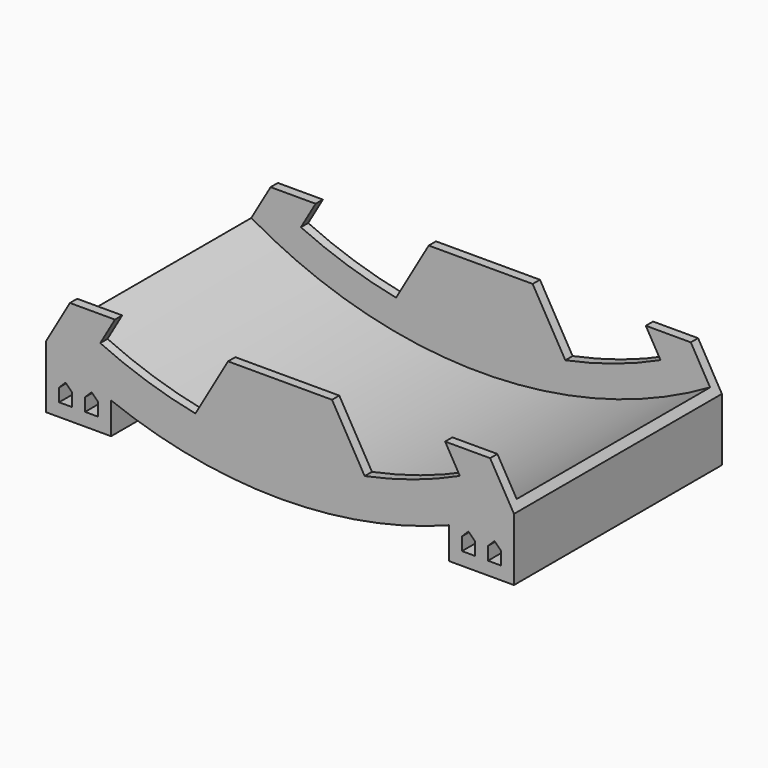
from build123d import *

# Parameters (mm, degrees)
F1_DEPTH  = 127
F2_T      = 4.445
F3_R      = 9.525
F4_DEPTH  = 127
F6_DEPTH  = 127
F8_DEPTH  = 154.94
F10_DEPTH = 4.445
F14_DEPTH = 127


# Not quite as in the source:
# - a shell that OpenCascade refuses in one call is made with other operations: the cavity is built on its own and cut out


with BuildPart() as f1:
    # F0 (on Front) → F1 (new body)
    with BuildSketch(Plane.XZ):
        with BuildLine():
            Line((-19.05, -32.9955678842), (-114.3, -197.9734073051))
            ThreePointArc((-114.3, -197.9734073051), (0, -228.6), (114.3, -197.9734073051))
            Line((114.3, -197.9734073051), (19.05, -32.9955678842))
            ThreePointArc((19.05, -32.9955678842), (32.9955678842, -19.05), (38.1, 0))
            ThreePointArc((38.1, 0), (0, 38.1), (-38.1, 0))
            ThreePointArc((-38.1, 0), (-32.9955678842, -19.05), (-19.05, -32.9955678842))
        make_face()
    extrude(amount=F1_DEPTH)

    # F2: shell of thickness 4.445, made by hand


with BuildPart() as f2_core1:
    # F2_t2: copy of F1
    add(f1.part)

    # the walls: a layer under each face that stays
    f2_faces = [f2_core1.faces().sort_by_distance(p)[0] for p in [
        (0, -127, -95.25),
        (0, 0, -95.25),
        (0, -63.5, -228.6),
        (-32.9955678842, -63.5, -19.05),
    ]]
    thicken(f2_faces, amount=-F2_T, mode=Mode.SUBTRACT)


with BuildPart() as f1_1:
    add(f1.part)

    # what is left inside the walls is the cavity
    f2_cavity = [f2_core1.part.solids().sort_by_distance(p)[0] for p in [
        (0, -122.51055, -136.736667),
    ]]
    add(f2_cavity, mode=Mode.SUBTRACT)

    # F3 (on face) → F4 (cut, through all)
    with BuildSketch(Plane.XZ.offset(127)):
        with BuildLine():
            Line((-50.6196632626, -125.7758286329), (-87.8433632626, -190.2491682786))
            ThreePointArc((-87.8433632626, -190.2491682786), (-48.4057129805, -203.8825383667), (-7.0486462544, -209.4314185741))
            Line((-7.0486462544, -209.4314185741), (-7.0486462544, -169.3468456411))
            Line((-7.0486462544, -169.3468456411), (-50.6196632626, -125.7758286329))
        make_face()
        with BuildLine():
            Line((87.8433632626, -190.2491682786), (50.6196632626, -125.7758286329))
            Line((50.6196632626, -125.7758286329), (7.0486462544, -169.3468456411))
            Line((7.0486462544, -169.3468456411), (7.0486462544, -209.4314185741))
            ThreePointArc((7.0486462544, -209.4314185741), (48.4057129805, -203.8825383667), (87.8433632626, -190.2491682786))
        make_face()
        with BuildLine():
            Line((44.2696632626, -114.7773060049), (7.0486462544, -50.3086134373))
            Line((7.0486462544, -50.3086134373), (7.0486462544, -125.901221947))
            ThreePointArc((7.0486462544, -125.901221947), (11.356209976, -128.3041542134), (14.9024469628, -131.7324762409))
            Line((14.9024469628, -131.7324762409), (44.2696632626, -114.7773060049))
        make_face()
        with BuildLine():
            Line((-7.0486462544, -125.901221947), (-7.0486462544, -50.3086134373))
            Line((-7.0486462544, -50.3086134373), (-44.2696632626, -114.7773060049))
            Line((-44.2696632626, -114.7773060049), (-14.9024469628, -131.7324762409))
            ThreePointArc((-14.9024469628, -131.7324762409), (-11.356209976, -128.3041542134), (-7.0486462544, -125.901221947))
        make_face()
        Circle(F3_R)
    extrude(amount=-F4_DEPTH, mode=Mode.SUBTRACT)

    # F5 (on Front) → F6 (join, through all)
    with BuildSketch(Plane.XZ):
        with BuildLine():
            ThreePointArc((114.3, -197.9734073051), (59.1660337104, -220.8106438897), (0, -228.6))
            Line((0, -228.6), (114.3, -228.6))
            Line((114.3, -228.6), (114.3, -197.9734073051))
        make_face()
        Polygon((95.25, -222.25), (88.9, -222.25), (88.9, -215.9), (92.075, -212.725), (95.25, -215.9), align=None, mode=Mode.SUBTRACT)
        Polygon((107.95, -215.9), (107.95, -222.25), (101.6, -222.25), (101.6, -215.9), (104.775, -212.725), align=None, mode=Mode.SUBTRACT)
        with BuildLine():
            Line((-114.3, -228.6), (0, -228.6))
            ThreePointArc((0, -228.6), (-59.1660337104, -220.8106438897), (-114.3, -197.9734073051))
            Line((-114.3, -197.9734073051), (-114.3, -228.6))
        make_face()
        Polygon((-104.775, -212.725), (-101.6, -215.9), (-101.6, -222.25), (-107.95, -222.25), (-107.95, -215.9), align=None, mode=Mode.SUBTRACT)
        Polygon((-92.075, -212.725), (-88.9, -215.9), (-88.9, -222.25), (-95.25, -222.25), (-95.25, -215.9), align=None, mode=Mode.SUBTRACT)
    extrude(amount=F6_DEPTH)

    # F7 (on Front) → F8 (cut)
    with BuildSketch(Plane.XZ):
        Polygon((-155.1303118467, -177.8), (0, -177.8), (122.5007101893, -177.8), (122.5007101893, 99.952660501), (-155.1303118467, 97.6831391454), align=None)
    extrude(amount=F8_DEPTH, mode=Mode.SUBTRACT)

    # F9 (on face) → F10 (join, through all)
    with BuildSketch(Plane(origin=(0, 0, 0), x_dir=(-1, 0, 0), z_dir=(0, 1, 0))):
        with BuildLine():
            ThreePointArc((-41.3518280797, -205.4293767076), (-65.0419791249, -199.2002596673), (-87.8433632626, -190.2491682786))
            Line((-87.8433632626, -190.2491682786), (-80.6558326058, -177.8))
            Line((-80.6558326058, -177.8), (-102.6528778619, -177.8))
            Line((-102.6528778619, -177.8), (-114.3, -197.9734073051))
            Line((-114.3, -197.9734073051), (-114.3, -228.6))
            Line((-114.3, -228.6), (114.3, -228.6))
            Line((114.3, -228.6), (114.3, -197.9734073051))
            Line((114.3, -197.9734073051), (102.6528778619, -177.8))
            Line((102.6528778619, -177.8), (80.6558326058, -177.8))
            Line((80.6558326058, -177.8), (87.8433632626, -190.2491682786))
            ThreePointArc((87.8433632626, -190.2491682786), (65.0419791249, -199.2002596673), (41.3518280797, -205.4293767076))
            ThreePointArc((41.3518280797, -205.4293767076), (24.2828244592, -208.1382880113), (7.0486462544, -209.4314185741))
            Line((7.0486462544, -209.4314185741), (7.0486462544, -177.8))
            Line((7.0486462544, -177.8), (0, -177.8))
            Line((0, -177.8), (-7.0486462544, -177.8))
            Line((-7.0486462544, -177.8), (-7.0486462544, -209.4314185741))
            ThreePointArc((-7.0486462544, -209.4314185741), (-24.2828244592, -208.1382880113), (-41.3518280797, -205.4293767076))
        make_face()
        Polygon((-107.95, -222.25), (-107.95, -215.9), (-104.775, -212.725), (-101.6, -215.9), (-101.6, -222.25), align=None, mode=Mode.SUBTRACT)
        Polygon((-88.9, -215.9), (-88.9, -222.25), (-95.25, -222.25), (-95.25, -215.9), (-92.075, -212.725), align=None, mode=Mode.SUBTRACT)
        Polygon((88.9, -215.9), (92.075, -212.725), (95.25, -215.9), (95.25, -222.25), (88.9, -222.25), align=None, mode=Mode.SUBTRACT)
        Polygon((101.6, -222.25), (101.6, -215.9), (104.775, -212.725), (107.95, -215.9), (107.95, -222.25), align=None, mode=Mode.SUBTRACT)
        with BuildLine():
            Line((-25.4, -177.8), (-41.3518280797, -205.4293767076))
            ThreePointArc((-41.3518280797, -205.4293767076), (-24.2828244592, -208.1382880113), (-7.0486462544, -209.4314185741))
            Line((-7.0486462544, -209.4314185741), (-7.0486462544, -177.8))
            Line((-7.0486462544, -177.8), (-25.4, -177.8))
        make_face()
        with BuildLine():
            Line((25.4, -177.8), (7.0486462544, -177.8))
            Line((7.0486462544, -177.8), (7.0486462544, -209.4314185741))
            ThreePointArc((7.0486462544, -209.4314185741), (24.2828244592, -208.1382880113), (41.3518280797, -205.4293767076))
            Line((41.3518280797, -205.4293767076), (25.4, -177.8))
        make_face()
    extrude(amount=-F10_DEPTH)

    # F12: F1 across plane


with BuildPart() as f1_2:
    add(f1_1.part)
    add(f1_1.part.mirror(Plane(origin=(0, -63.5, -104.9820841324), x_dir=(1, 0, 0), z_dir=(0, -1, 0))))

    # F13 (on face) → F14 (cut, through all)
    with BuildSketch(Plane.XZ.offset(127)):
        with BuildLine():
            ThreePointArc((0, -228.6), (-41.9894094809, -224.7105905191), (-82.55, -213.1747112113))
            Line((-82.55, -213.1747112113), (-82.55, -228.6))
            Line((-82.55, -228.6), (0, -228.6))
        make_face()
        with BuildLine():
            ThreePointArc((82.55, -213.1747112113), (41.9894094809, -224.7105905191), (0, -228.6))
            Line((0, -228.6), (82.55, -228.6))
            Line((82.55, -228.6), (82.55, -213.1747112113))
        make_face()
    extrude(amount=-F14_DEPTH, mode=Mode.SUBTRACT)


solid = f1_2.part
